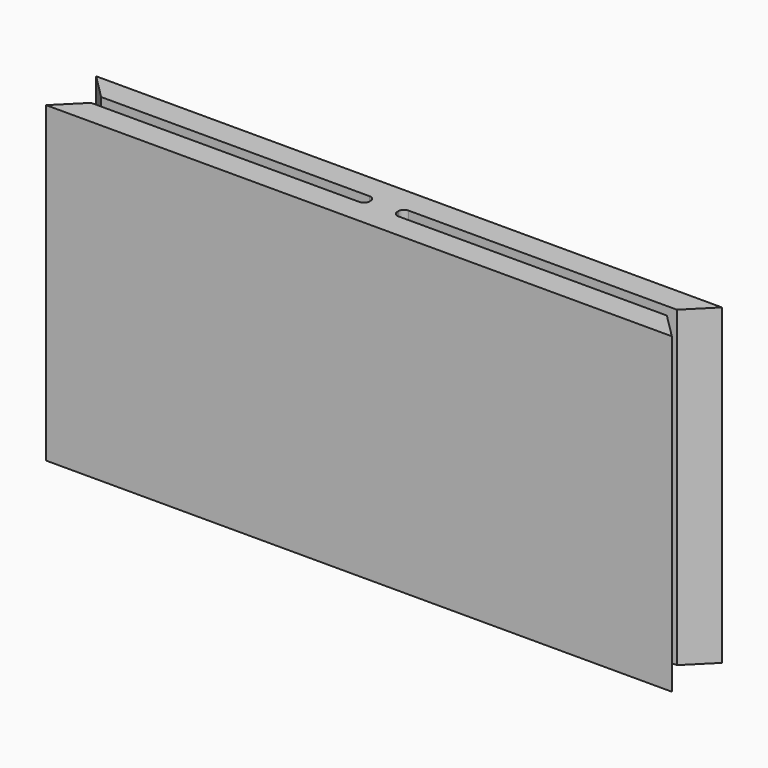
from build123d import *

# Parameters (mm, degrees)
F1_DEPTH    = 10
F2_T1_DEPTH = 14.1146927807
F3_R        = 0.18


# Not quite as in the source:
# - a fillet or chamfer that OpenCascade refuses, or shapes differently, is made with other operations: its cross-section is extruded or revolved along the edge and cut away or added


with BuildPart() as f1:
    # F0 (on Top) → F1 (new body)
    with BuildSketch(Plane.XY):
        Polygon((10, 0.2012402692), (10, 1), (0.4449767875, 1), (-0.4449767875, 1), (-10, 1), (-10, 0.2012402692), (-0.4449767875, 0.2012402692), (-0.4449767875, -0.2012402692), (-10, -0.2012402692), (-10, -1), (-0.4449767875, -1), (0.4449767875, -1), (10, -1), (10, -0.2012402692), (0.4449767875, -0.2012402692), (0.4449767875, 0.2012402692), align=None)
    extrude(amount=F1_DEPTH)

    # F2: chamfer of 0.8 on 4 edges, made by hand

    # F2_s2 → F2_t1 (cut)
    with BuildSketch(Plane.XY.offset(-2.0573463904)):
        Polygon((-10, -1.0012402692), (-9.2, -0.2012402692), (-10, -0.2012402692), align=None)
        Polygon((-9.2, 0.2012402692), (-10, 1.0012402692), (-10, 0.2012402692), align=None)
        Polygon((9.2, -0.2012402692), (10, -1.0012402692), (10, -0.2012402692), align=None)
        Polygon((10, 1.0012402692), (9.2, 0.2012402692), (10, 0.2012402692), align=None)
    extrude(amount=F2_T1_DEPTH, mode=Mode.SUBTRACT)

    # F3
    f3_edges = [f1.edges().sort_by_distance(p)[0] for p in [
        (-0.444977, -0.20124, 5),
        (-0.444977, 0.20124, 5),
        (0.444977, 0.20124, 5),
        (0.444977, -0.20124, 5),
    ]]
    fillet(f3_edges, radius=F3_R)


solid = f1.part
